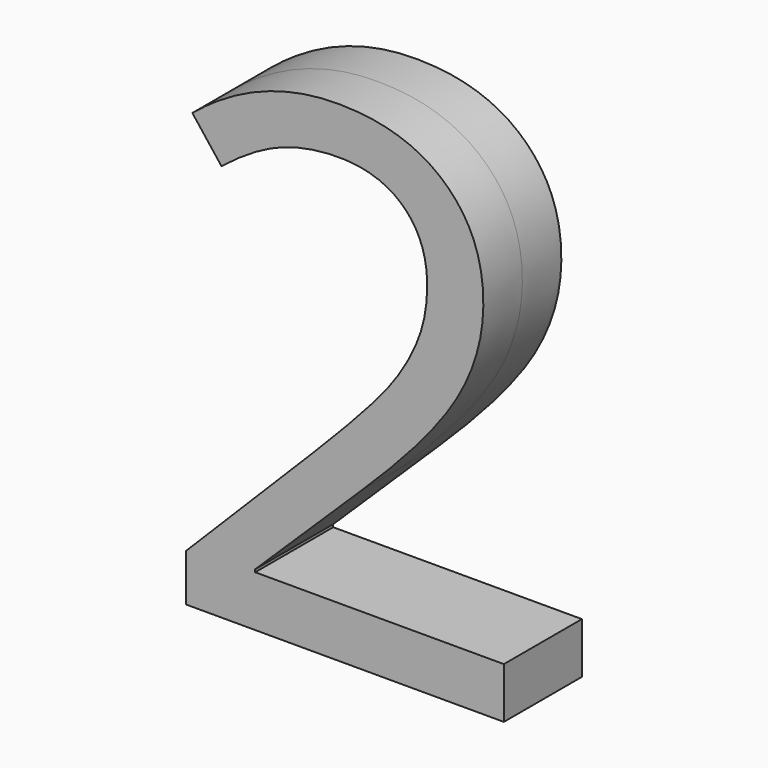
from build123d import *

# Parameters (mm, degrees)
F0_TEXT_SIZE  = 138.8888888889
F1_DEPTH      = 10
F1_DEPTH_BACK = 10


# Not quite as in the source:
# - Text() gives the source's letters only with a copy of the font that has no kerning and outlines rounded to 1/6400 em; it was checked with that copy


with BuildPart() as f1:
    # F0 (on Front) → F1 (new body, two sides)
    with BuildSketch(Plane.XZ) as f1_sk:
        with Locations((-40.4839409722, 0)):
            Text('2', F0_TEXT_SIZE, font='Open Sans', text_align=(TextAlign.LEFT, TextAlign.BOTTOM))
    extrude(amount=F1_DEPTH)
    extrude(f1_sk.sketch, amount=-F1_DEPTH_BACK)


solid = f1.part
